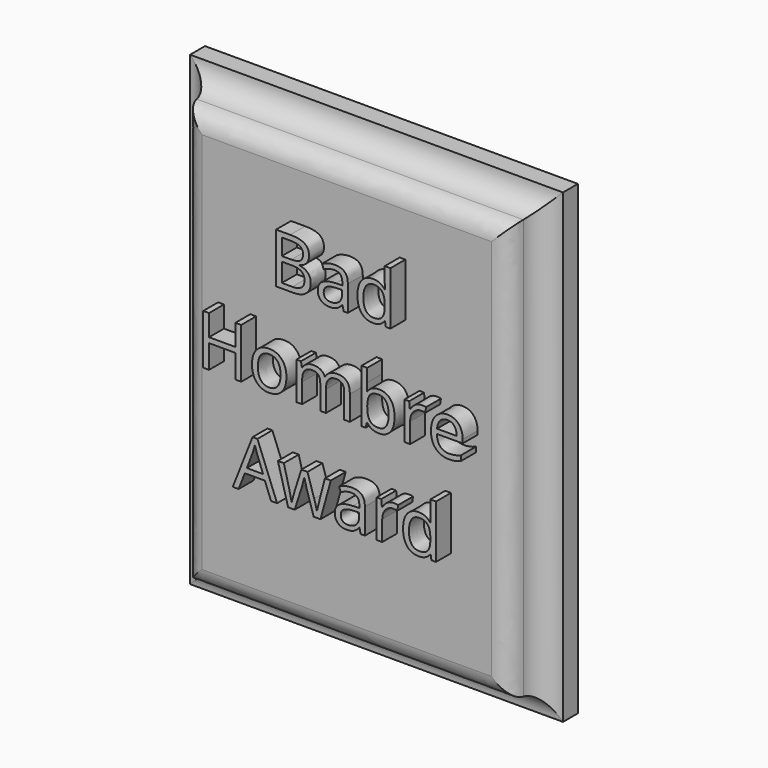
from build123d import *

# Parameters (mm, degrees)
F0_W         = 101.6
F0_H         = 127
F1_DEPTH     = 15.24
F2_W         = 101.6
F2_H         = 127
F2_W_2       = 88.9
F2_H_2       = 114.3
F3_DEPTH     = 10.16
F4_R         = 6.34999
F5_R         = 5.08
F6_TEXT_SIZE = 19.0863505003
F7_DEPTH     = 5.08


# Not quite as in the source:
# - a fillet or chamfer is up to 0.001 mm smaller than in the source, because OpenCascade refuses the exact size
# - Text() gives the source's letters only with a copy of the font that has no kerning and outlines rounded to 1/6400 em; it was checked with that copy


with BuildPart() as f1:
    # F0 (on Front) → F1 (new body)
    with BuildSketch(Plane.XZ):
        with Locations((-50.8, 63.5)):
            Rectangle(F0_W, F0_H)
    extrude(amount=F1_DEPTH)

    # F2 (on face) → F3 (cut)
    with BuildSketch(Plane.XZ.offset(15.24)):
        with Locations((-50.8, 63.5)):
            Rectangle(F2_W, F2_H)
        with Locations((-50.8, 63.5)):
            Rectangle(F2_W_2, F2_H_2, mode=Mode.SUBTRACT)
    extrude(amount=-F3_DEPTH, mode=Mode.SUBTRACT)

    # F4 (radius 6.35 in the source; OpenCascade refuses exactly that, so slightly less here)
    f4_edges = [f1.edges().sort_by_distance(p)[0] for p in [
        (-50.8, -5.08, 120.65),
        (-6.35, -5.08, 63.5),
        (-95.25, -5.08, 63.5),
        (-50.8, -5.08, 6.35),
    ]]
    fillet(f4_edges, radius=F4_R)

    # F5
    f5_edges = [f1.edges().sort_by_distance(p)[0] for p in [
        (-6.35, -15.24, 63.5),
        (-50.8, -15.24, 6.35),
        (-95.25, -15.24, 63.5),
        (-50.8, -15.24, 120.65),
    ]]
    fillet(f5_edges, radius=F5_R)

    # F6 (on face) → F7 (join)
    with BuildSketch(Plane.XZ.offset(15.24)):
        with Locations((-67.862899123, 89.1986023141)):
            Text('Bad', F6_TEXT_SIZE, font='Open Sans', text_align=(TextAlign.LEFT, TextAlign.BOTTOM))
        with Locations((-87.7007746743, 63.2411656337)):
            Text('Hombre', F6_TEXT_SIZE, font='Open Sans', text_align=(TextAlign.LEFT, TextAlign.BOTTOM))
        with Locations((-77.7818368987, 37.2837289533)):
            Text('Award', F6_TEXT_SIZE, font='Open Sans', text_align=(TextAlign.LEFT, TextAlign.BOTTOM))
    extrude(amount=F7_DEPTH)


solid = f1.part
